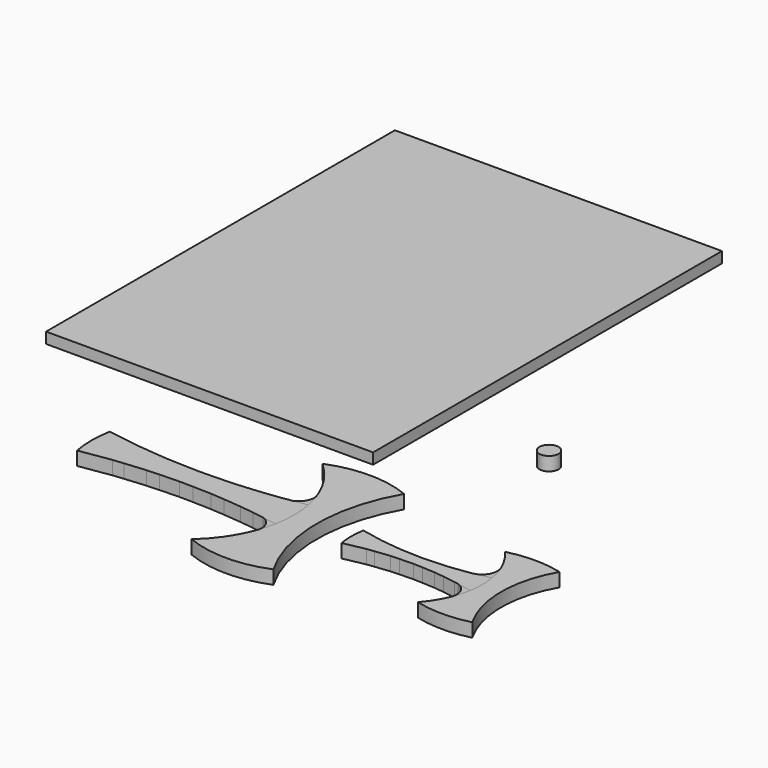
from build123d import *

# Parameters (mm, degrees)
F1_DEPTH  = 6.35
F2_R      = 7.112
F4_DEPTH  = 6.35
F5_R      = 7.239
F6_DEPTH  = 6.35
F7_DEPTH  = 6.35
F8_DEPTH  = 6.35
F9_DEPTH  = 6.35
F10_W     = 152.4
F10_H     = 203.2
F11_DEPTH = 5.08
F12_R     = 4.445
F13_DEPTH = 6.35


# Not quite as in the source:
# - a length typed as a fraction of an inch, garbled in the dataset ("3 / 203.2 mm" for 3/8 in), is restored


with BuildPart() as f1:
    # F0 (on Top) → F1 (new body)
    with BuildSketch(Plane.XY):
        with BuildLine():
            ThreePointArc((-28.1519998261, -9.525), (-27.2510416505, 0), (-28.1519998261, 9.525))
            ThreePointArc((-28.1519998261, 9.525), (-74.400999913, 5.2789388898), (-120.65, 9.525))
            ThreePointArc((-120.65, 9.525), (-121.5509581755, 0), (-120.65, -9.525))
            ThreePointArc((-120.65, -9.525), (-74.400999913, -5.2789388898), (-28.1519998261, -9.525))
        make_face()
        with BuildLine():
            ThreePointArc((-6.35, -38.1), (-16.5588642316, 0), (-6.35, 38.1))
            ThreePointArc((-6.35, 38.1), (-25.4, 41.8071396069), (-44.45, 38.1))
            ThreePointArc((-44.45, 38.1), (-33.9239678598, 25.1682609385), (-28.1519998261, 9.525))
            ThreePointArc((-28.1519998261, 9.525), (-27.2510416505, 0), (-28.1519998261, -9.525))
            ThreePointArc((-28.1519998261, -9.525), (-33.9239678598, -25.1682609385), (-44.45, -38.1))
            ThreePointArc((-44.45, -38.1), (-25.4, -41.8071396069), (-6.35, -38.1))
        make_face()
    extrude(amount=F1_DEPTH)

    # F2
    f2_edges = [f1.edges().sort_by_distance(p)[0] for p in [
        (-28.152, 9.525, 3.175),
        (-28.152, -9.525, 3.175),
    ]]
    fillet(f2_edges, radius=F2_R)


with BuildPart() as f4:
    # F3 (on Top) → F4 (new body)
    with BuildSketch(Plane.XY):
        with BuildLine():
            ThreePointArc((59.9690433084, -6.35), (60.5019366858, 0), (59.9690433084, 6.35))
            ThreePointArc((59.9690433084, 6.35), (29.9845216542, 2.7595963091), (0, 6.35))
            ThreePointArc((0, 6.35), (-0.5328933773, 0), (0, -6.35))
            ThreePointArc((0, -6.35), (29.9845216542, -2.7595963091), (59.9690433084, -6.35))
        make_face()
        with BuildLine():
            ThreePointArc((76.2, -25.4), (69.3940905122, 0), (76.2, 25.4))
            ThreePointArc((76.2, 25.4), (63.5, 27.0131115032), (50.8, 25.4))
            ThreePointArc((50.8, 25.4), (56.7323391914, 16.5237242714), (59.9690433084, 6.35))
            ThreePointArc((59.9690433084, 6.35), (60.5019366858, 0), (59.9690433084, -6.35))
            ThreePointArc((59.9690433084, -6.35), (56.7323391914, -16.5237242714), (50.8, -25.4))
            ThreePointArc((50.8, -25.4), (63.5, -27.0131115032), (76.2, -25.4))
        make_face()
    extrude(amount=F4_DEPTH)

    # F5
    f5_edges = [f4.edges().sort_by_distance(p)[0] for p in [
        (59.969043, -6.35, 3.175),
        (59.969043, 6.35, 3.175),
    ]]
    fillet(f5_edges, radius=F5_R)


with BuildPart() as f6:
    # F0 (on Top) → F6 (new body)
    with BuildSketch(Plane.XY):
        with BuildLine():
            ThreePointArc((-6.35, -38.1), (-16.5588642316, 0), (-6.35, 38.1))
            ThreePointArc((-6.35, 38.1), (-25.4, 41.8071396069), (-44.45, 38.1))
            ThreePointArc((-44.45, 38.1), (-33.9239678598, 25.1682609385), (-28.1519998261, 9.525))
            ThreePointArc((-28.1519998261, 9.525), (-27.2510416505, 0), (-28.1519998261, -9.525))
            ThreePointArc((-28.1519998261, -9.525), (-33.9239678598, -25.1682609385), (-44.45, -38.1))
            ThreePointArc((-44.45, -38.1), (-25.4, -41.8071396069), (-6.35, -38.1))
        make_face()
    extrude(amount=F6_DEPTH)


with BuildPart() as f7:
    # F0 (on Top) → F7 (new body)
    with BuildSketch(Plane.XY):
        with BuildLine():
            ThreePointArc((-28.1519998261, -9.525), (-27.2510416505, 0), (-28.1519998261, 9.525))
            ThreePointArc((-28.1519998261, 9.525), (-74.400999913, 5.2789388898), (-120.65, 9.525))
            ThreePointArc((-120.65, 9.525), (-121.5509581755, 0), (-120.65, -9.525))
            ThreePointArc((-120.65, -9.525), (-74.400999913, -5.2789388898), (-28.1519998261, -9.525))
        make_face()
    extrude(amount=F7_DEPTH)


with BuildPart() as f8:
    # F3 (on Top) → F8 (new body)
    with BuildSketch(Plane.XY):
        with BuildLine():
            ThreePointArc((76.2, -25.4), (69.3940905122, 0), (76.2, 25.4))
            ThreePointArc((76.2, 25.4), (63.5, 27.0131115032), (50.8, 25.4))
            ThreePointArc((50.8, 25.4), (56.7323391914, 16.5237242714), (59.9690433084, 6.35))
            ThreePointArc((59.9690433084, 6.35), (60.5019366858, 0), (59.9690433084, -6.35))
            ThreePointArc((59.9690433084, -6.35), (56.7323391914, -16.5237242714), (50.8, -25.4))
            ThreePointArc((50.8, -25.4), (63.5, -27.0131115032), (76.2, -25.4))
        make_face()
    extrude(amount=F8_DEPTH)


with BuildPart() as f9:
    # F3 (on Top) → F9 (new body)
    with BuildSketch(Plane.XY):
        with BuildLine():
            ThreePointArc((59.9690433084, -6.35), (60.5019366858, 0), (59.9690433084, 6.35))
            ThreePointArc((59.9690433084, 6.35), (29.9845216542, 2.7595963091), (0, 6.35))
            ThreePointArc((0, 6.35), (-0.5328933773, 0), (0, -6.35))
            ThreePointArc((0, -6.35), (29.9845216542, -2.7595963091), (59.9690433084, -6.35))
        make_face()
    extrude(amount=F9_DEPTH)


with BuildPart() as f11:
    # F10 (on Top) → F11 (new body)
    with BuildSketch(Plane.XY):
        with Locations((-113.3361747384, 160.0966391325)):
            Rectangle(F10_W, F10_H)
    extrude(amount=F11_DEPTH)


with BuildPart() as f13:
    # F12 (on Top) → F13 (new body)
    with BuildSketch(Plane.XY):
        with Locations((13.3899739012, 97.8238731623)):
            Circle(F12_R)
    extrude(amount=F13_DEPTH)


solid = Compound([f1.part, f4.part, f6.part, f7.part, f8.part, f9.part, f11.part, f13.part])
